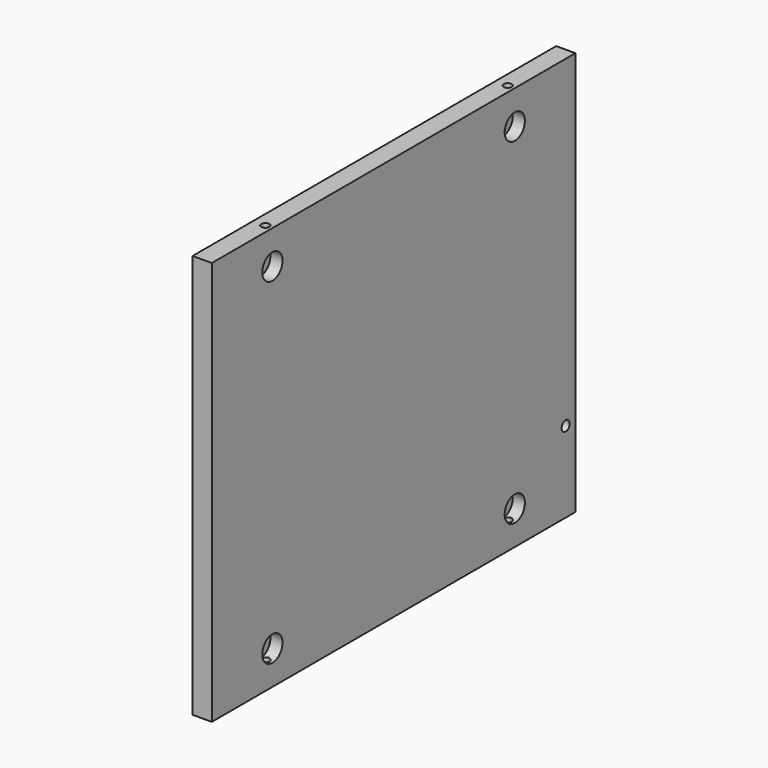
from build123d import *

# Parameters (mm, degrees)
F0_W     = 450
F0_H     = 400
F1_DEPTH = 19
F2_R     = 12.5
F3_DEPTH = 12
F5_D     = 8
F5_DEPTH = 22
F5_TIP   = 2.4034424761
F7_D     = 10
F7_DEPTH = 13
F7_TIP   = 3.0043030951


# Not quite as in the source:
# - a pattern or mirror of a feature is missing from the dataset's text; its kind, count and spacing are read off the source's solid


with BuildPart() as f1:
    # F0 (on Right) → F1 (new body)
    with BuildSketch(Plane.YZ):
        Rectangle(F0_W, F0_H)
    extrude(amount=-F1_DEPTH)

    # F2 (on face) → F3 (cut)
    with BuildSketch(Plane.YZ):
        with Locations((-150, -166.5)):
            Circle(F2_R)
        with Locations((150, -166.5)):
            Circle(F2_R)
        with Locations((-150, 166.5)):
            Circle(F2_R)
        with Locations((150, 166.5)):
            Circle(F2_R)
    extrude(amount=-F3_DEPTH, mode=Mode.SUBTRACT)

    # F5
    with Locations(Plane.XY.offset(200)):
        with Locations((-7, 150), (-7, -150)):
            f5 = Hole(F5_D / 2, depth=F5_DEPTH)
            with Locations((0, 0, -(F5_DEPTH + F5_TIP / 2))):  # 118° drill point
                Cone(0, F5_D / 2, F5_TIP, mode=Mode.SUBTRACT)

    # F5_copies: F5 across plane
    add(f5.mirror(Plane(origin=(0, 0, 2.1e-05), x_dir=(-1, 0, 0), z_dir=(0, 0, -1))), mode=Mode.SUBTRACT)

    # F7
    with Locations(Plane.YZ):
        with Locations((213, -120)):
            Hole(F7_D / 2, depth=F7_DEPTH)
            with Locations((0, 0, -(F7_DEPTH + F7_TIP / 2))):  # 118° drill point
                Cone(0, F7_D / 2, F7_TIP, mode=Mode.SUBTRACT)


solid = f1.part
